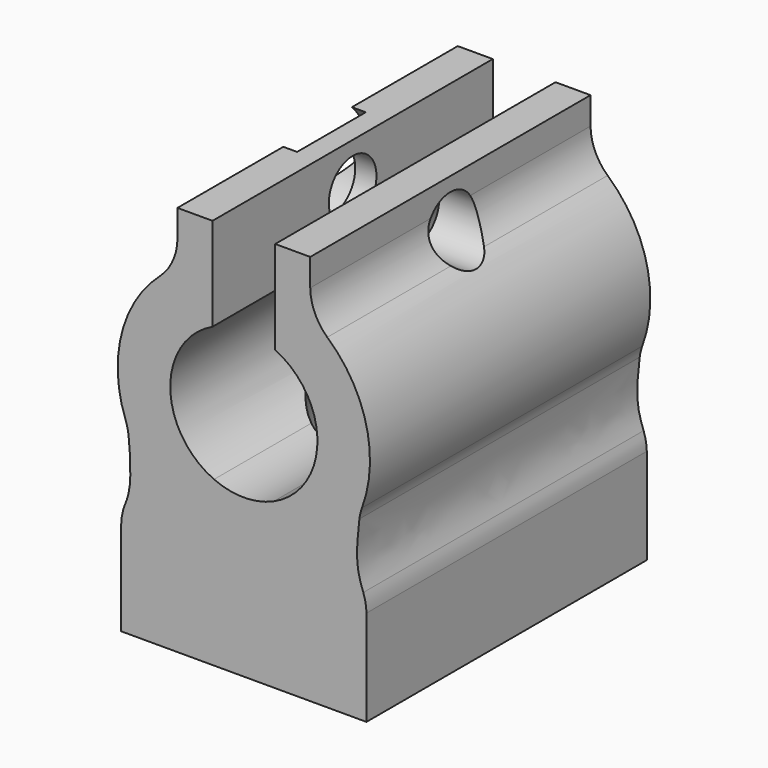
from build123d import *

# Parameters (mm, degrees)
F1_DEPTH     = 20
F2_R         = 3.5
F2_R_2       = 1.7
F3_DEPTH     = 4
F4_DEPTH     = 25
F5_T1_DEPTH  = 20
F5_T6_DEPTH  = 12.1022846539
F5_S7_R      = 1.7
F5_T8_DEPTH  = 8
F5_T12_DEPTH = 12.1022846539
F5_S13_R     = 1.7
F5_T14_DEPTH = 8
F5_T18_DEPTH = 10.2630041323
F5_S19_R     = 3.5
F5_T20_DEPTH = 7
F5_T24_DEPTH = 10.2630041323
F5_S25_R     = 3.5
F5_T26_DEPTH = 7
F5_T27_DEPTH = 23.3663915102
F5_T29_DEPTH = 22.9020360067
F6_R         = 3.5
F6_R_2       = 1.7
F7_DEPTH     = 12
F8_DEPTH     = 12
F9_DEPTH     = 6
F10_DEPTH    = 10


# Not quite as in the source:
# - a fillet or chamfer that OpenCascade refuses, or shapes differently, is made with other operations: its cross-section is extruded or revolved along the edge and cut away or added


with BuildPart() as f1:
    # F0 (on Front) → F1 (new body)
    with BuildSketch(Plane.XZ):
        with BuildLine():
            ThreePointArc((-1.7, -3.8405728739), (-4.1997120304, -0.0491819207), (-1.7894736842, 3.7997084011))
            Line((-1.7894736842, 3.7997084011), (-1.7894736842, 9.1220820965))
            Line((-1.7894736842, 9.1220820965), (-3.7894736842, 9.1220820965))
            Line((-3.7894736842, 9.1220820965), (-3.7894736842, 6.1220820965))
            ThreePointArc((-3.7894736842, 6.1220820965), (-6.8557776995, 2.199616361), (-6.6439040907, -2.7746240166))
            add(Edge.make_bspline(
                [(-6.6356726702, -2.7942527112), (-6.6390399212, -2.7803089062), (-6.6413283577, -2.7774058988), (-6.6439040907, -2.7746240166)],
                knots=[0.9532514843, 0.9532514843, 0.9532514843, 0.9532514843, 1, 1, 1, 1], degree=3))
            add(Edge.make_bspline(
                [(-7, -7.2), (-6.7795680226, -6.7700727801), (-6.2785456929, -5.7974600377), (-6.5973790049, -2.9528269921), (-6.6356726702, -2.7942527112)],
                knots=[0, 0, 0, 0, 0.4216094964, 0.9532514843, 0.9532514843, 0.9532514843, 0.9532514843], degree=3))
            Line((-7, -7.2), (-7, -13.2))
            Line((-7, -13.2), (-1.7, -13.2))
            Line((-1.7, -13.2), (-1.7, -4.2))
            Line((-1.7, -4.2), (-1.7, -3.8405728739))
        make_face()
        with BuildLine():
            ThreePointArc((1.7, -3.8405728739), (0, -4.2), (-1.7, -3.8405728739))
            Line((-1.7, -3.8405728739), (-1.7, -4.2))
            Line((-1.7, -4.2), (-1.7, -13.2))
            Line((-1.7, -13.2), (1.7, -13.2))
            Line((1.7, -13.2), (1.7, -4.2))
            Line((1.7, -4.2), (1.7, -3.8405728739))
        make_face()
        with BuildLine():
            ThreePointArc((1.7894736842, 3.7997084011), (4.1997120304, -0.0491819207), (1.7, -3.8405728739))
            Line((1.7, -3.8405728739), (1.7, -4.2))
            Line((1.7, -4.2), (1.7, -13.2))
            Line((1.7, -13.2), (7, -13.2))
            Line((7, -13.2), (7, -7.2))
            add(Edge.make_bspline(
                [(7, -7.2), (6.7871491537, -6.6864508711), (6.3058923114, -5.5253136877), (6.5175995563, -3.7720698099), (6.6356726702, -2.7942527112)],
                knots=[0, 0, 0, 0, 0.4422811845, 1, 1, 1, 1], degree=3))
            ThreePointArc((6.6356726702, -2.7942527112), (6.8590214848, 2.1894803656), (3.7894736842, 6.1220820965))
            Line((3.7894736842, 6.1220820965), (3.7894736842, 9.1220820965))
            Line((3.7894736842, 9.1220820965), (1.7894736842, 9.1220820965))
            Line((1.7894736842, 9.1220820965), (1.7894736842, 3.7997084011))
        make_face()
        with BuildLine():
            add(Edge.make_bspline(
                [(-6.6356726702, -2.7942527112), (-6.6390399212, -2.7803089062), (-6.6413283577, -2.7774058988), (-6.6439040907, -2.7746240166)],
                knots=[0.9532514843, 0.9532514843, 0.9532514843, 0.9532514843, 1, 1, 1, 1], degree=3))
            ThreePointArc((-6.6439040907, -2.7746240166), (-6.6397956338, -2.7844414056), (-6.6356726702, -2.7942527112))
        make_face()
    extrude(amount=F1_DEPTH)

    # F2 (on face) → F3 (cut)
    with BuildSketch(Plane(origin=(-7, 0, 0), x_dir=(0, -1, 0), z_dir=(-1, 0, 0))):
        with Locations((10, 6.622)):
            Circle(F2_R)
        with Locations((10, 6.622)):
            Circle(F2_R_2, mode=Mode.SUBTRACT)
    extrude(amount=-F3_DEPTH, mode=Mode.SUBTRACT)

    # F2 (on face) → F4 (cut)
    with BuildSketch(Plane(origin=(-7, 0, 0), x_dir=(0, -1, 0), z_dir=(-1, 0, 0))):
        with Locations((10, 6.622)):
            Circle(F2_R_2)
    extrude(amount=-F4_DEPTH, mode=Mode.SUBTRACT)

    # F5: fillet of radius 3 on 8 edges, made by hand

    # F5_s2 → F5_t1 (join)
    with BuildSketch(Plane.XZ):
        with BuildLine():
            ThreePointArc((-6.7483493849, -2.5087886996), (-6.6395606645, -2.8691274316), (-6.5767127025, -3.2402461743))
            Line((-6.5767127025, -3.2402461743), (-6.2781272304, -3.2087696206))
            ThreePointArc((-6.2781272304, -3.2087696206), (-6.304537605, -2.9799785061), (-6.343821894, -2.723774473))
            Line((-6.343821894, -2.723774473), (-6.3589651198, -2.6777323732))
            ThreePointArc((-6.3589651198, -2.6777323732), (-6.4145893512, -2.5416001874), (-6.466927581, -2.4041663985))
            Line((-6.466927581, -2.4041663985), (-6.7483493849, -2.5087886996))
        make_face()
        with BuildLine():
            ThreePointArc((6.5887317904, -3.1834061265), (6.6509501418, -2.8334452349), (6.754091056, -2.4932898281))
            Line((6.754091056, -2.4932898281), (6.4724298111, -2.3893138658))
            ThreePointArc((6.4724298111, -2.3893138658), (6.4175024363, -2.534235691), (6.3589651198, -2.6777323732))
            Line((6.3589651198, -2.6777323732), (6.3375979172, -2.7582596669))
            ThreePointArc((6.3375979172, -2.7582596669), (6.3141276632, -2.9530960278), (6.290534619, -3.1484417941))
            Line((6.290534619, -3.1484417941), (6.5887317904, -3.1834061265))
        make_face()
    extrude(amount=F5_T1_DEPTH)


with BuildPart() as f5_tool4:
    # F5_s5 → F5_t6 (new body)
    with BuildSketch(Plane.XZ.offset(7.8977153461)):
        with BuildLine():
            ThreePointArc((4.792775332, 5.3724803189), (4.0514647707, 6.385428811), (3.7890736842, 7.6129290813))
            Line((3.7890736842, 7.6129290813), (3.4888336842, 7.6129290813))
            ThreePointArc((3.4888336842, 7.6129290813), (3.4892336842, 6.8675055889), (3.4892336842, 6.1220820965))
            Line((3.4892336842, 6.1220820965), (3.6314526316, 5.8667912731))
            ThreePointArc((3.6314526316, 5.8667912731), (4.1279416848, 5.5287236777), (4.5929054968, 5.1484354427))
            Line((4.5929054968, 5.1484354427), (4.792775332, 5.3724803189))
        make_face()
    extrude(amount=F5_T6_DEPTH)

    # F5_s7 → F5_t8 (cut, symmetric)
    with BuildSketch(Plane.YZ.offset(4.1)):
        with Locations((-10, 6.622)):
            Circle(F5_S7_R)
    extrude(amount=F5_T8_DEPTH, both=True, mode=Mode.SUBTRACT)


with BuildPart() as f1_1:
    add(f1.part)

    # F5_t3: union F5_tool4
    add(f5_tool4.part)


with BuildPart() as f5_tool10:
    # F5_s11 → F5_t12 (new body)
    with BuildSketch(Plane.XZ):
        with BuildLine():
            ThreePointArc((4.792775332, 5.3724803189), (4.0514647707, 6.385428811), (3.7890736842, 7.6129290813))
            Line((3.7890736842, 7.6129290813), (3.4888336842, 7.6129290813))
            ThreePointArc((3.4888336842, 7.6129290813), (3.4892336842, 6.8675055889), (3.4892336842, 6.1220820965))
            Line((3.4892336842, 6.1220820965), (3.6314526316, 5.8667912731))
            ThreePointArc((3.6314526316, 5.8667912731), (4.1279416848, 5.5287236777), (4.5929054968, 5.1484354427))
            Line((4.5929054968, 5.1484354427), (4.792775332, 5.3724803189))
        make_face()
    extrude(amount=F5_T12_DEPTH)

    # F5_s13 → F5_t14 (cut, symmetric)
    with BuildSketch(Plane.YZ.offset(4.1)):
        with Locations((-10, 6.622)):
            Circle(F5_S13_R)
    extrude(amount=F5_T14_DEPTH, both=True, mode=Mode.SUBTRACT)


with BuildPart() as f1_2:
    add(f1_1.part)

    # F5_t9: union F5_tool10
    add(f5_tool10.part)


with BuildPart() as f5_tool16:
    # F5_s17 → F5_t18 (new body)
    with BuildSketch(Plane.XZ):
        with BuildLine():
            ThreePointArc((-3.7890736842, 7.6129290813), (-4.0514647707, 6.385428811), (-4.792775332, 5.3724803189))
            Line((-4.792775332, 5.3724803189), (-4.5929054968, 5.1484354427))
            ThreePointArc((-4.5929054968, 5.1484354427), (-4.1279416848, 5.5287236777), (-3.6314526316, 5.8667912731))
            Line((-3.6314526316, 5.8667912731), (-3.4892336842, 6.1220820965))
            ThreePointArc((-3.4892336842, 6.1220820965), (-3.4892336842, 6.8675055889), (-3.4888336842, 7.6129290813))
            Line((-3.4888336842, 7.6129290813), (-3.7890736842, 7.6129290813))
        make_face()
    extrude(amount=F5_T18_DEPTH)

    # F5_s19 → F5_t20 (cut, symmetric)
    with BuildSketch(Plane.YZ.offset(-4.1)):
        with Locations((-10, 6.622)):
            Circle(F5_S19_R)
    extrude(amount=F5_T20_DEPTH, both=True, mode=Mode.SUBTRACT)


with BuildPart() as f1_3:
    add(f1_2.part)

    # F5_t15: union F5_tool16
    add(f5_tool16.part)


with BuildPart() as f5_tool22:
    # F5_s23 → F5_t24 (new body)
    with BuildSketch(Plane.XZ.offset(9.7369958677)):
        with BuildLine():
            ThreePointArc((-4.792775332, 5.3724803189), (-4.0514647707, 6.385428811), (-3.7890736842, 7.6129290813))
            Line((-3.7890736842, 7.6129290813), (-3.4888336842, 7.6129290813))
            ThreePointArc((-3.4888336842, 7.6129290813), (-3.4892336842, 6.8675055889), (-3.4892336842, 6.1220820965))
            Line((-3.4892336842, 6.1220820965), (-3.6314526316, 5.8667912731))
            ThreePointArc((-3.6314526316, 5.8667912731), (-4.1279416848, 5.5287236777), (-4.5929054968, 5.1484354427))
            Line((-4.5929054968, 5.1484354427), (-4.792775332, 5.3724803189))
        make_face()
    extrude(amount=F5_T24_DEPTH)

    # F5_s25 → F5_t26 (cut, symmetric)
    with BuildSketch(Plane.YZ.offset(-4.1)):
        with Locations((-10, 6.622)):
            Circle(F5_S25_R)
    extrude(amount=F5_T26_DEPTH, both=True, mode=Mode.SUBTRACT)


with BuildPart() as f1_4:
    add(f1_3.part)

    # F5_t21: union F5_tool22
    add(f5_tool22.part)

    # F5_s28 → F5_t27 (cut)
    with BuildSketch(Plane.XZ.offset(-1.6831957551)):
        with BuildLine():
            ThreePointArc((-7.0004, -7.8732781832), (-6.9416848839, -7.2824101234), (-6.7678360085, -6.7146521667))
            Line((-6.7678360085, -6.7146521667), (-7.0448196093, -6.5987895651))
            ThreePointArc((-7.0448196093, -6.5987895651), (-7.148871707, -6.8283644641), (-7.2671697753, -7.0630169034))
            Line((-7.2671697753, -7.0630169034), (-7.30024, -7.2))
            ThreePointArc((-7.30024, -7.2), (-7.30024, -7.5366390916), (-7.30064, -7.8732781832))
            Line((-7.30064, -7.8732781832), (-7.0004, -7.8732781832))
        make_face()
    extrude(amount=F5_T27_DEPTH, mode=Mode.SUBTRACT)

    # F5_s30 → F5_t29 (cut)
    with BuildSketch(Plane.XZ.offset(-1.4510180034)):
        with BuildLine():
            ThreePointArc((6.8044646756, -6.7135604089), (6.9510099307, -7.2380620544), (7.0004, -7.7804070635))
            Line((7.0004, -7.7804070635), (7.30064, -7.7804070635))
            ThreePointArc((7.30064, -7.7804070635), (7.30024, -7.4902035318), (7.30024, -7.2))
            Line((7.30024, -7.2), (7.277360411, -7.0850423555))
            ThreePointArc((7.277360411, -7.0850423555), (7.178454263, -6.8447161783), (7.0851111432, -6.6068757434))
            Line((7.0851111432, -6.6068757434), (6.8044646756, -6.7135604089))
        make_face()
    extrude(amount=F5_T29_DEPTH, mode=Mode.SUBTRACT)

    # F6 (on face) → F7 (cut)
    with BuildSketch(Plane(origin=(0, 0, -13.2), x_dir=(1, 0, 0), z_dir=(0, 0, -1))):
        with Locations((0, 10)):
            Circle(F6_R)
        with Locations((0, 10)):
            Circle(F6_R_2, mode=Mode.SUBTRACT)
    extrude(amount=-F7_DEPTH, mode=Mode.SUBTRACT)

    # F8 (cut): a face of the model
    f8_faces = [f1_4.faces().sort_by_distance(p)[0] for p in [
        (0, -10, -13.2),
    ]]
    extrude(f8_faces, amount=-F8_DEPTH, mode=Mode.SUBTRACT)

    # F6 (on face) → F9 (join)
    with BuildSketch(Plane(origin=(0, 0, -13.2), x_dir=(1, 0, 0), z_dir=(0, 0, -1))):
        with Locations((0, 10)):
            Circle(F6_R)
        with Locations((0, 10)):
            Circle(F6_R_2, mode=Mode.SUBTRACT)
    extrude(amount=-F9_DEPTH)

    # F0 (on Front) → F10 (cut)
    with BuildSketch(Plane.XZ):
        with BuildLine():
            ThreePointArc((1.7, -3.8405728739), (0, -4.2), (-1.7, -3.8405728739))
            Line((-1.7, -3.8405728739), (-1.7, -4.2))
            Line((-1.7, -4.2), (-1.7, -13.2))
            Line((-1.7, -13.2), (1.7, -13.2))
            Line((1.7, -13.2), (1.7, -4.2))
            Line((1.7, -4.2), (1.7, -3.8405728739))
        make_face()
    extrude(amount=F10_DEPTH, mode=Mode.SUBTRACT)


solid = f1_4.part
